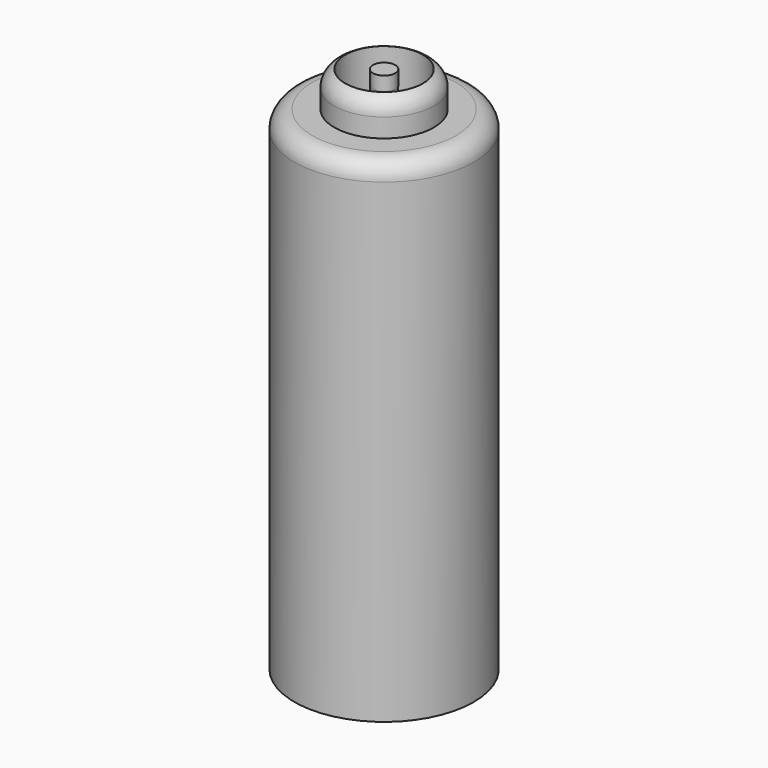
from build123d import *


# Not quite as in the source:
# - a fillet or chamfer that OpenCascade refuses, or shapes differently, is made with other operations: its cross-section is extruded or revolved along the edge and cut away or added


with BuildPart() as f1:
    # F0 (on Front) → F1 (revolve)
    with BuildSketch(Plane.XZ):
        Polygon((25.4, -69.85), (25.4, 69.85), (14.1084063798, 69.85), (14.1084063798, 79.8223763704), (11.0044367611, 79.8223763704), (11.0044367611, 75.8906826377), (11.0044367611, 64.0955939889), (22.3856568336, 64.0955939889), (22.3856568336, -66.8919235468), (1.6925277887, -66.8919235468), (3.1410455704, 75.8906826377), (3.1410455704, 79.8223763704), (0, 79.8223763704), (0, 0), (0, -69.85), align=None)
    revolve(axis=Axis((0, 0, 39.9111881852), (0, 0, -1)))

    # F2: fillet of radius 5.08 on 2 edges, made by hand

    # F2_s1 → F2_t2 (revolve, cut)
    with BuildSketch(Plane.XZ):
        with BuildLine():
            ThreePointArc((25.4004, 64.7690343146), (23.9121024484, 68.3621024484), (20.3190343146, 69.8504))
            Line((20.3190343146, 69.8504), (20.3190343146, 70.3585365685))
            ThreePointArc((20.3190343146, 70.3585365685), (22.8595171573, 70.3581365685), (25.4, 70.3581365685))
            Line((25.4, 70.3581365685), (25.9081365685, 69.85))
            ThreePointArc((25.9081365685, 69.85), (25.9081365685, 67.3095171573), (25.9085365685, 64.7690343146))
            Line((25.9085365685, 64.7690343146), (25.4004, 64.7690343146))
        make_face()
    revolve(axis=Axis((0, 0, 69.85), (0, 0, -1)), mode=Mode.SUBTRACT)

    # F2_s3 → F2_t4 (revolve, cut)
    with BuildSketch(Plane.XZ):
        with BuildLine():
            ThreePointArc((14.1088063798, 75.1418102884), (13.2622316021, 77.9501591266), (11.0045924005, 79.8227448489))
            Line((11.0045924005, 79.8227448489), (11.2023075712, 80.2908383049))
            ThreePointArc((11.2023075712, 80.2908383049), (12.5564993902, 80.330512939), (14.1084063798, 80.330512939))
            Line((14.1084063798, 80.330512939), (14.6165429484, 79.8223763704))
            ThreePointArc((14.6165429484, 79.8223763704), (14.6165429484, 77.4820933294), (14.6169429484, 75.1418102884))
            Line((14.6169429484, 75.1418102884), (14.1088063798, 75.1418102884))
        make_face()
    revolve(axis=Axis((0, 0, 79.8223763704), (0, 0, -1)), mode=Mode.SUBTRACT)


solid = f1.part
